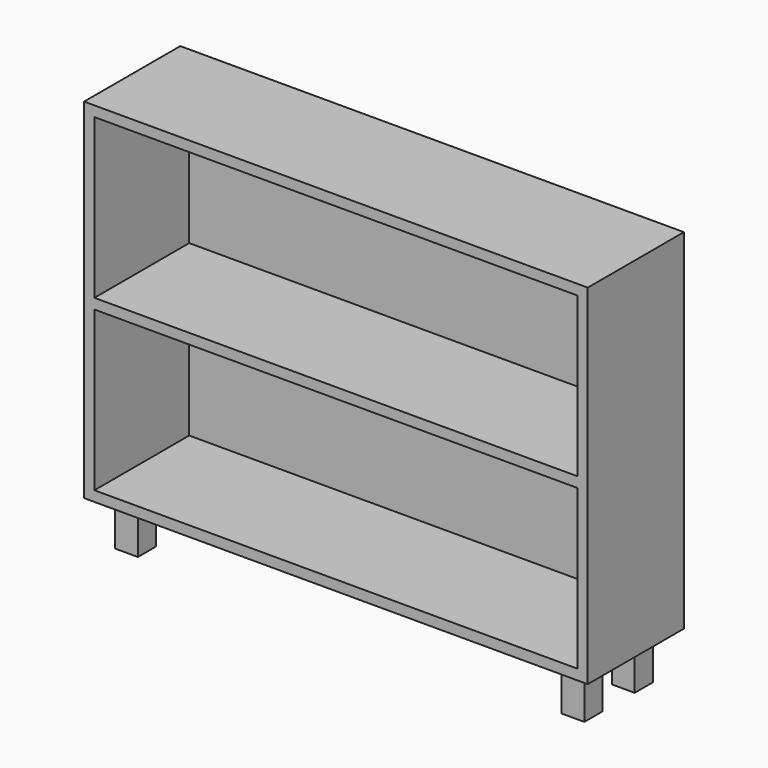
from build123d import *

# Parameters (mm, degrees)
F0_W     = 880
F0_H     = 690
F1_DEPTH = 210
F2_W     = 880
F2_H     = 210
F2_W_2   = 40
F2_H_2   = 40
F3_DEPTH = 80
F4_W     = 844
F4_H     = 278
F5_DEPTH = 207


# Not quite as in the source:
# - a feature names something its author has since deleted; it is built from what else it names


with BuildPart() as f1:
    # F0 (on Front) → F1 (new body)
    with BuildSketch(Plane.XZ):
        with Locations((402.0964676142, 312.2104381025)):
            Rectangle(F0_W, F0_H)
    extrude(amount=F1_DEPTH)

    # F2 (on face) → F3 (cut)
    with BuildSketch(Plane(origin=(0, 0, -32.7895618975), x_dir=(1, 0, 0), z_dir=(0, 0, -1))):
        with Locations((402.0964676142, 105)):
            Rectangle(F2_W, F2_H)
        with Locations((12.0964676142, 50)):
            Rectangle(F2_W_2, F2_H_2, mode=Mode.SUBTRACT)
        with Locations((792.0964676142, 50)):
            Rectangle(F2_W_2, F2_H_2, mode=Mode.SUBTRACT)
        with Locations((12.0964676142, 160)):
            Rectangle(F2_W_2, F2_H_2, mode=Mode.SUBTRACT)
        with Locations((792.0964676142, 160)):
            Rectangle(F2_W_2, F2_H_2, mode=Mode.SUBTRACT)
    extrude(amount=-F3_DEPTH, mode=Mode.SUBTRACT)

    # F4 (on face) → F5 (cut, through all)
    with BuildSketch(Plane.XZ.offset(210)):
        with Locations((402.0964676142, 500.2104381025)):
            Rectangle(F4_W, F4_H)
        with Locations((402.0964676142, 204.2104381025)):
            Rectangle(F4_W, F4_H)
    extrude(amount=-F5_DEPTH, mode=Mode.SUBTRACT)


solid = f1.part
